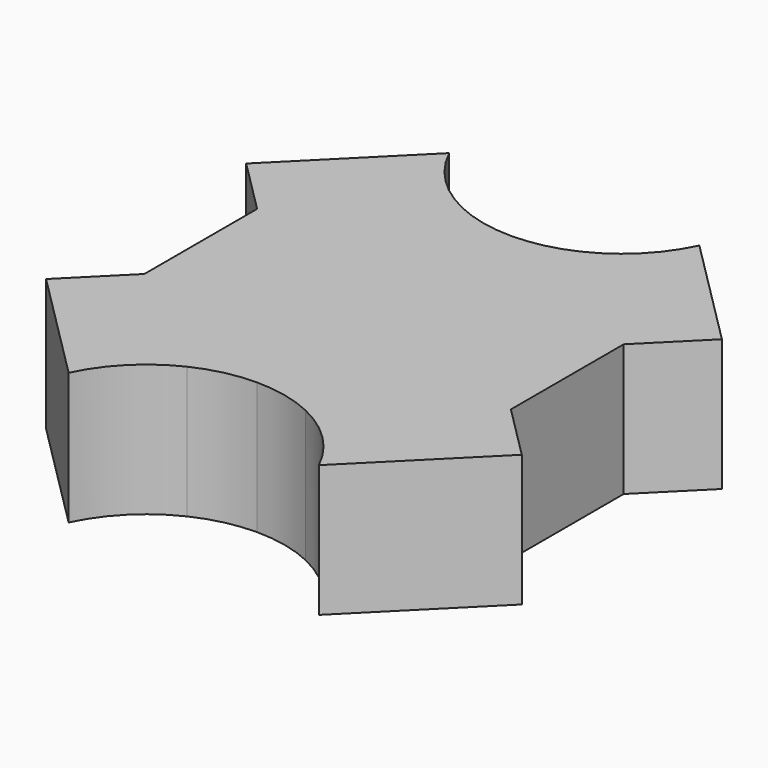
from build123d import *

# Parameters (mm, degrees)
F1_DEPTH = 15.24


# Not quite as in the source:
# - a feature names something its author has since deleted; it is built from what else it names


with BuildPart() as f1:
    # F0 (on Top) → F1 (new body)
    with BuildSketch(Plane.XY):
        with BuildLine():
            ThreePointArc((-6.8469626463, 19.8860116913), (-11.313708499, 23.0332541473), (-14.4609509549, 27.5))
            Line((-14.4609509549, 27.5), (-27.5, 14.4609509549))
            Line((-27.5, 14.4609509549), (-21.1890490451, 8.15))
            Line((-21.1890490451, 8.15), (-13.0390490451, 0))
            Line((-13.0390490451, 0), (0, 13.0390490451))
            Line((0, 13.0390490451), (-6.8469626463, 19.8860116913))
        make_face()
        Polygon((-13.0390490451, 0), (-21.1890490451, 8.15), (-21.1890490451, -8.15), align=None)
        with BuildLine():
            Line((14.4609509549, -27.5), (27.5, -14.4609509549))
            Line((27.5, -14.4609509549), (21.1890490451, -8.15))
            Line((21.1890490451, -8.15), (13.0390490451, 0))
            Line((13.0390490451, 0), (0, -13.0390490451))
            Line((0, -13.0390490451), (6.8469626463, -19.8860116913))
            ThreePointArc((6.8469626463, -19.8860116913), (11.313708499, -23.0332541473), (14.4609509549, -27.5))
        make_face()
        Polygon((13.0390490451, 0), (0, 13.0390490451), (0, 0), (0, -13.0390490451), align=None)
        Polygon((0, 0), (0, 13.0390490451), (-13.0390490451, 0), (0, -13.0390490451), align=None)
        with BuildLine():
            Line((27.5, 14.4609509549), (14.4609509549, 27.5))
            ThreePointArc((14.4609509549, 27.5), (11.313708499, 23.0332541473), (6.8469626463, 19.8860116913))
            Line((6.8469626463, 19.8860116913), (0, 13.0390490451))
            Line((0, 13.0390490451), (13.0390490451, 0))
            Line((13.0390490451, 0), (21.1890490451, 8.15))
            Line((21.1890490451, 8.15), (27.5, 14.4609509549))
        make_face()
        Polygon((21.1890490451, -8.15), (21.1890490451, 8.15), (13.0390490451, 0), align=None)
        with BuildLine():
            Line((0, -13.0390490451), (-6.8469626463, -19.8860116913))
            ThreePointArc((-6.8469626463, -19.8860116913), (-3.5089018739, -18.7364659329), (0, -18.3469626463))
            Line((0, -18.3469626463), (0, -13.0390490451))
        make_face()
        with BuildLine():
            Line((0, 13.0390490451), (6.8469626463, 19.8860116913))
            ThreePointArc((6.8469626463, 19.8860116913), (3.5089018739, 18.7364659329), (0, 18.3469626463))
            Line((0, 18.3469626463), (0, 13.0390490451))
        make_face()
        with BuildLine():
            ThreePointArc((0, 18.3469626463), (-3.5089018739, 18.7364659329), (-6.8469626463, 19.8860116913))
            Line((-6.8469626463, 19.8860116913), (0, 13.0390490451))
            Line((0, 13.0390490451), (0, 18.3469626463))
        make_face()
        with BuildLine():
            Line((6.8469626463, -19.8860116913), (0, -13.0390490451))
            Line((0, -13.0390490451), (0, -18.3469626463))
            ThreePointArc((0, -18.3469626463), (3.5089018739, -18.7364659329), (6.8469626463, -19.8860116913))
        make_face()
        with BuildLine():
            Line((-21.1890490451, -8.15), (-27.5, -14.4609509549))
            Line((-27.5, -14.4609509549), (-14.4609509549, -27.5))
            ThreePointArc((-14.4609509549, -27.5), (-11.313708499, -23.0332541473), (-6.8469626463, -19.8860116913))
            Line((-6.8469626463, -19.8860116913), (0, -13.0390490451))
            Line((0, -13.0390490451), (-13.0390490451, 0))
            Line((-13.0390490451, 0), (-21.1890490451, -8.15))
        make_face()
    extrude(amount=F1_DEPTH)


solid = f1.part
